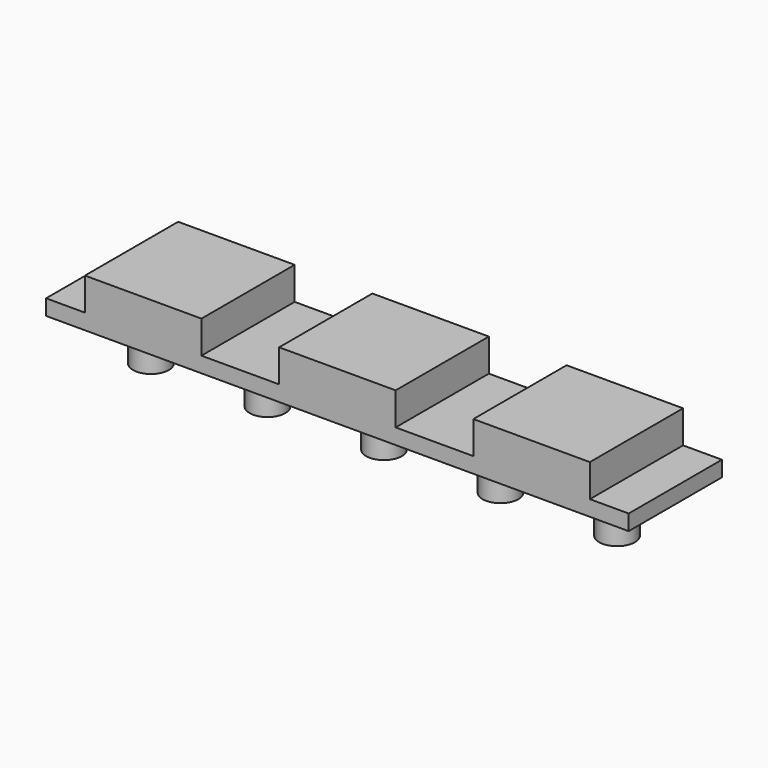
from build123d import *

# Parameters (mm, degrees)
F0_W     = 15
F0_H     = 15
F0_R     = 2.3
F1_DEPTH = 2
F2_DEPTH = 8
F4_DEPTH = 7.5
F5_START = 5.5
F3_W     = 11
F3_H     = 2.2
F5_DEPTH = 2


# Not quite as in the source:
# - a feature names something its author has since deleted; it is built from what else it names


with BuildPart() as f1:
    # F0 (on Top) → F1 (new body)
    with BuildSketch(Plane.XY):
        with Locations((-30, 0)):
            Rectangle(F0_W, F0_H)
        with Locations((-30, 0)):
            Circle(F0_R, mode=Mode.SUBTRACT)
        with Locations((-15, 0)):
            Rectangle(F0_W, F0_H)
        with Locations((-15, 0)):
            Circle(F0_R, mode=Mode.SUBTRACT)
        Rectangle(F0_W, F0_H)
        Circle(F0_R, mode=Mode.SUBTRACT)
        with Locations((15, 0)):
            Rectangle(F0_W, F0_H)
        with Locations((15, 0)):
            Circle(F0_R, mode=Mode.SUBTRACT)
        with Locations((30, 0)):
            Rectangle(F0_W, F0_H)
        with Locations((30, 0)):
            Circle(F0_R, mode=Mode.SUBTRACT)
    extrude(amount=-F1_DEPTH)

    # F0 (on Top) → F2 (join)
    with BuildSketch(Plane.XY):
        with Locations((-15, 0)):
            Circle(F0_R)
        with Locations((-30, 0)):
            Circle(F0_R)
        Circle(F0_R)
        with Locations((15, 0)):
            Circle(F0_R)
        with Locations((30, 0)):
            Circle(F0_R)
    extrude(amount=-F2_DEPTH)

    # F3 (on Front) → F4 (join, symmetric)
    with BuildSketch(Plane.XZ):
        Polygon((-32.5, 4.2), (-32.5, 0), (-30.5, 0), (-30.5, 2.2), (-19.5, 2.2), (-19.5, 0), (-17.5, 0), (-17.5, 4.2), align=None)
        Polygon((5.5, 2.2), (5.5, 0), (7.5, 0), (7.5, 4.2), (-7.5, 4.2), (-7.5, 0), (-5.5, 0), (-5.5, 2.2), align=None)
        Polygon((30.5, 2.2), (30.5, 0), (32.5, 0), (32.5, 4.2), (17.5, 4.2), (17.5, 0), (19.5, 0), (19.5, 2.2), align=None)
    extrude(amount=F4_DEPTH, both=True)

    # F3 (on Front) → F5 (join)
    with BuildSketch(Plane.XZ.offset(F5_START)):
        with Locations((-25, 1.1)):
            Rectangle(F3_W, F3_H)
        with Locations((0, 1.1)):
            Rectangle(F3_W, F3_H)
        with Locations((25, 1.1)):
            Rectangle(F3_W, F3_H)
    extrude(amount=F5_DEPTH)


solid = f1.part
